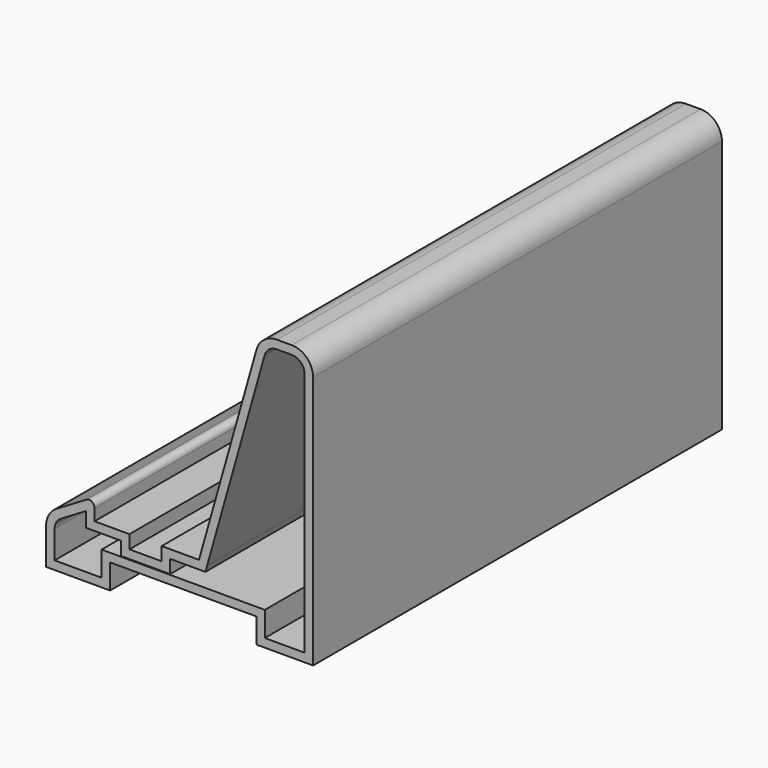
from build123d import *

# Parameters (mm, degrees)
F1_DEPTH    = 152.4
F2_T        = 2.54
F2_T3_DEPTH = 157.48


# Not quite as in the source:
# - a shell that OpenCascade refuses in one call is made with other operations: the cavity is built on its own and cut out


with BuildPart() as f1:
    # F0 (on Front) → F1 (new body)
    with BuildSketch(Plane.XZ):
        with BuildLine():
            Line((-37.8300789744, -10.7009902054), (-48.2259040094, -10.7009902054))
            Line((-48.2259040094, -10.7009902054), (-48.2259040094, -7.2357404328))
            ThreePointArc((-48.2259040094, -7.2357404328), (-49.0552526275, -5.8106548767), (-50.7040085729, -5.8277371868))
            Line((-50.7040085729, -5.8277371868), (-59.5905011949, -11.123357617))
            ThreePointArc((-59.5905011949, -11.123357617), (-61.8609001823, -13.4412951055), (-62.6898407936, -16.578236805))
            Line((-62.6898407936, -16.578236805), (-62.6898407936, -27.3817684501))
            Line((-62.6898407936, -27.3817684501), (-43.5946621001, -27.3817684501))
            Line((-43.5946621001, -27.3817684501), (-43.5946621001, -19.9903684501))
            Line((-43.5946621001, -19.9903684501), (0, -19.9903684501))
            Line((0, -19.9903684501), (0, -27.3817684501))
            Line((0, -27.3817684501), (16.9334635139, -27.3817684501))
            Line((16.9334635139, -27.3817684501), (16.9334635139, 48.305941894))
            ThreePointArc((16.9334635139, 48.305941894), (15.0735915744, 52.7960699546), (10.5834635139, 54.655941894))
            Line((10.5834635139, 54.655941894), (6.1501904505, 54.655941894))
            ThreePointArc((6.1501904505, 54.655941894), (2.3177679163, 53.3690474153), (0.0387070827, 50.0299694591))
            Line((0.0387070827, 50.0299694591), (-17.0932790838, -10.7009902054))
            Line((-17.0932790838, -10.7009902054), (-28.2165445387, -10.7009902054))
            Line((-28.2165445387, -10.7009902054), (-28.2165445387, -14.6972788498))
            Line((-28.2165445387, -14.6972788498), (-37.8300789744, -14.6972788498))
            Line((-37.8300789744, -14.6972788498), (-37.8300789744, -10.7009902054))
        make_face()
    extrude(amount=F1_DEPTH)

    # F2: shell of thickness 2.54, made by hand


with BuildPart() as f2_core1:
    # F2_t2: copy of F1
    add(f1.part)

    # the walls: a layer under each face that stays
    f2_faces = [f2_core1.faces().sort_by_distance(p)[0] for p in [
        (-8.5272860005, -76.2, 19.6644896269),
        (-22.6549118113, -76.2, -10.7009902054),
        (-28.2165445387, -76.2, -12.6991345276),
        (-33.0233117566, -76.2, -14.6972788498),
        (-37.8300789744, -76.2, -12.6991345276),
        (-43.0279914919, -76.2, -10.7009902054),
        (-48.2259040094, -76.2, -8.9683653191),
        (-55.1472548839, -76.2, -8.4755474019),
        (-61.8609001823, -76.2, -13.4412951055),
        (-62.6898407936, -76.2, -21.9800026276),
        (-53.1422514468, -76.2, -27.3817684501),
        (-43.5946621001, -76.2, -23.6860684501),
        (-21.79733105, -76.2, -19.9903684501),
        (0, -76.2, -23.6860684501),
        (8.4667317569, -76.2, -27.3817684501),
        (16.9334635139, -76.2, 10.4620867219),
        (15.0735915744, -76.2, 52.7960699546),
        (8.3668269822, -76.2, 54.655941894),
        (2.3177679163, -76.2, 53.3690474153),
    ]]
    thicken(f2_faces, amount=-F2_T, mode=Mode.SUBTRACT)

    # F2_s4 → F2_t3 (cut)
    with BuildSketch(Plane.XZ.offset(-2.54)):
        Polygon((-17.1177250172, -10.6686940951), (-14.6486857366, -11.3906012314), (-15.1706738376, -13.2409902054), (-17.0932790838, -13.2409902054), align=None)
        Polygon((-28.2419445387, -14.6718788498), (-25.6765445387, -14.6972788498), (-25.6765445387, -17.2372788498), (-28.2165445387, -17.2372788498), align=None)
        Polygon((-37.8046789744, -14.6718788498), (-37.8300789744, -17.2372788498), (-40.3700789744, -17.2372788498), (-40.3700789744, -14.6972788498), align=None)
        Polygon((-48.2005040094, -10.6755902054), (-48.2259040094, -13.2409902054), (-50.7659040094, -13.2409902054), (-50.7659040094, -10.7009902054), align=None)
        Polygon((-43.5692621001, -20.0157684501), (-46.1346621001, -19.9903684501), (-46.1346621001, -17.4503684501), (-43.5946621001, -17.4503684501), align=None)
        Polygon((-0.0254, -20.0157684501), (0, -17.4503684501), (2.54, -17.4503684501), (2.54, -19.9903684501), align=None)
    extrude(amount=F2_T3_DEPTH, mode=Mode.SUBTRACT)


with BuildPart() as f1_1:
    add(f1.part)

    # what is left inside the walls is the cavity
    f2_cavity = [f2_core1.part.solids().sort_by_distance(p)[0] for p in [
        (14.368064, -101.6, 11.732087),
    ]]
    add(f2_cavity, mode=Mode.SUBTRACT)


solid = f1_1.part
